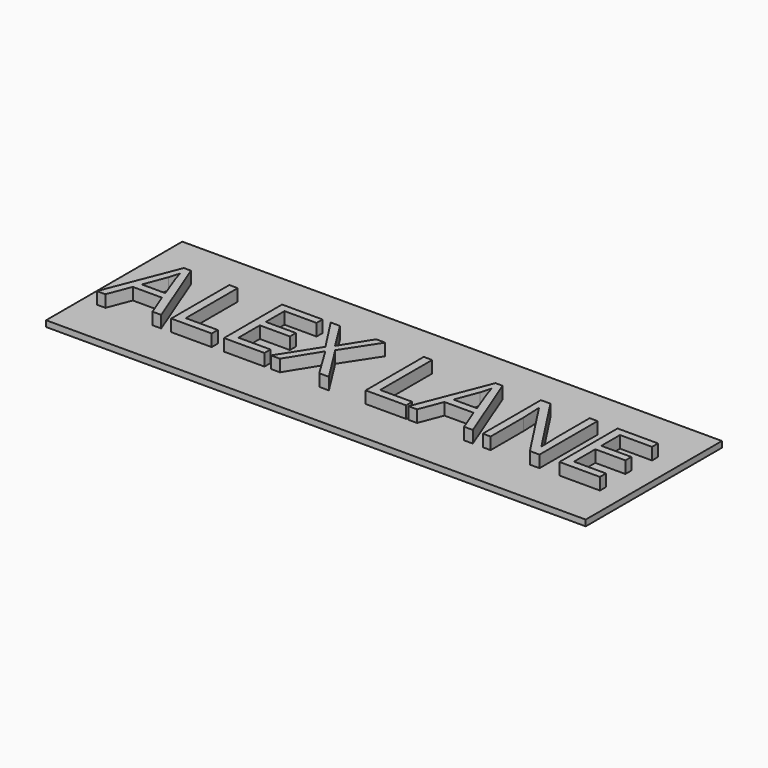
from build123d import *

# Parameters (mm, degrees)
F0_W         = 90
F0_H         = 28.3943
F1_DEPTH     = 1
F2_TEXT_SIZE = 16.9602494154
F3_DEPTH     = 2


# Not quite as in the source:
# - Text() gives the source's letters only with a copy of the font that has no kerning and outlines rounded to 1/6400 em; it was checked with that copy


with BuildPart() as f1:
    # F0 (on Top) → F1 (new body)
    with BuildSketch(Plane.XY):
        with Locations((45, 14.19715)):
            Rectangle(F0_W, F0_H)
    extrude(amount=F1_DEPTH)

    # F2 (on face) → F3 (join)
    with BuildSketch(Plane.XY.offset(1)):
        with Locations((2.4300092637, 7.5518882633)):
            Text('ALEX LANE', F2_TEXT_SIZE, font='Open Sans', text_align=(TextAlign.LEFT, TextAlign.BOTTOM))
    extrude(amount=F3_DEPTH)


solid = f1.part
